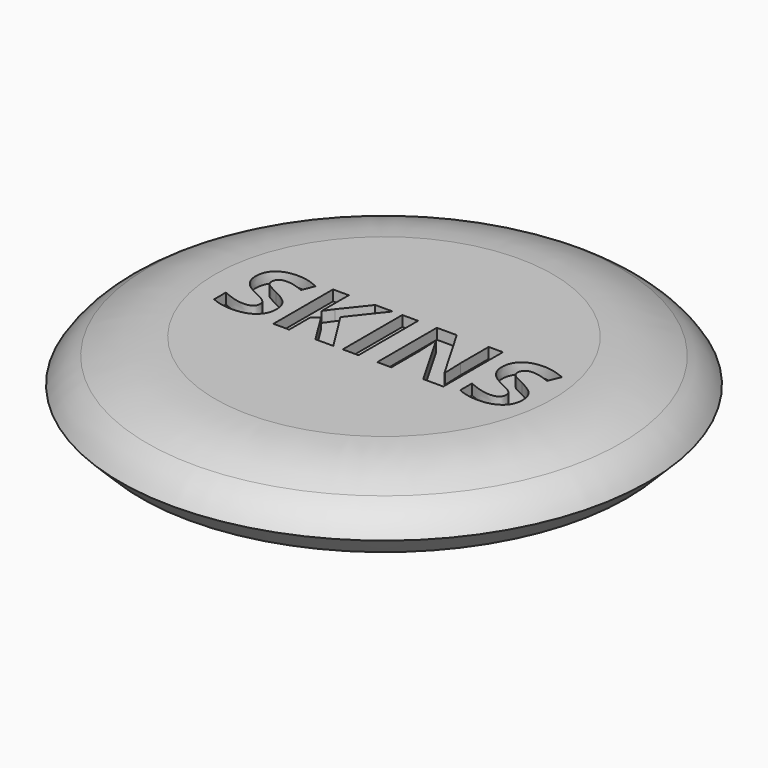
from build123d import *

# Parameters (mm, degrees)
F0_R         = 50
F1_DEPTH     = 12
F2_SIZE      = 4
F5_TEXT_SIZE = 19.7614991482
F6_DEPTH     = 2


# Not quite as in the source:
# - Text() gives the source's letters only with a copy of the font that has no kerning and outlines rounded to 1/6400 em; it was checked with that copy


with BuildPart() as f1:
    # F0 (on Top) → F1 (new body)
    with BuildSketch(Plane.XY):
        Circle(F0_R)
    extrude(amount=F1_DEPTH)

    # F2
    f2_edges = [f1.edges().sort_by_distance(p)[0] for p in [
        (-50, 0, 0),
    ]]
    chamfer(f2_edges, length=F2_SIZE)

    # F3 (on Front) → F4 (revolve, cut)
    with BuildSketch(Plane.XZ):
        with BuildLine():
            Line((-50, 12), (-50, 4))
            ThreePointArc((-50, 4), (-47.7685622075, 6.7523700981), (-44.8737123605, 8.7955783943))
            ThreePointArc((-44.8737123605, 8.7955783943), (-38.6245196568, 11.1517242015), (-32, 12))
            Line((-32, 12), (-50, 12))
        make_face()
    revolve(axis=Axis((0, 0, 32.4962362647), (0, 0, 1)), mode=Mode.SUBTRACT)

    # F5 (on face) → F6 (cut)
    with BuildSketch(Plane.XY.offset(12)):
        with Locations((-28, -7.0065842226)):
            Text('SKINS', F5_TEXT_SIZE, font='Open Sans', font_style=FontStyle.BOLD, text_align=(TextAlign.LEFT, TextAlign.BOTTOM))
    extrude(amount=-F6_DEPTH, mode=Mode.SUBTRACT)


solid = f1.part
